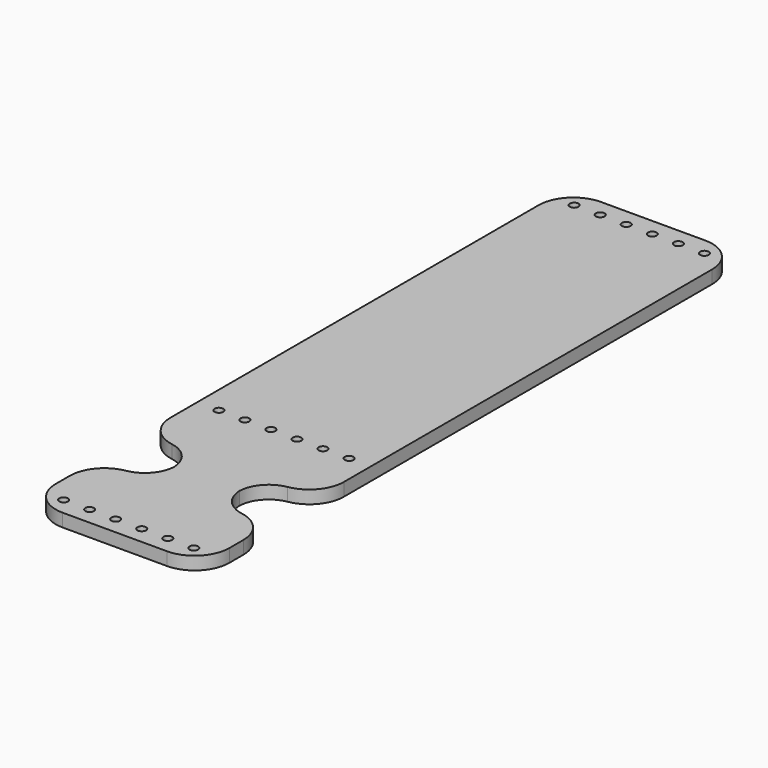
from build123d import *

# Parameters (mm, degrees)
F0_W        = 40
F0_H        = 155
F1_DEPTH    = 3
F2_W        = 12.5
F2_H        = 13
F3_DEPTH    = 3
F4_R        = 8
F5_T1_DEPTH = 3
F6_R        = 1
F7_DEPTH    = 3


# Not quite as in the source:
# - a fillet or chamfer that OpenCascade refuses, or shapes differently, is made with other operations: its cross-section is extruded or revolved along the edge and cut away or added


with BuildPart() as f1:
    # F0 (on Top) → F1 (new body)
    with BuildSketch(Plane.XY):
        Rectangle(F0_W, F0_H)
    extrude(amount=F1_DEPTH)

    # F2 (on face) → F3 (cut, through all)
    with BuildSketch(Plane.XY.offset(3)):
        with Locations((-13.75, -51)):
            Rectangle(F2_W, F2_H)
        with Locations((13.75, -51)):
            Rectangle(F2_W, F2_H)
    extrude(amount=-F3_DEPTH, mode=Mode.SUBTRACT)

    # F4
    f4_edges = [f1.edges().sort_by_distance(p)[0] for p in [
        (-20, -44.5, 1.5),
        (20, -44.5, 1.5),
        (20, -57.5, 1.5),
        (-20, -57.5, 1.5),
        (-20, -77.5, 1.5),
        (20, -77.5, 1.5),
        (-20, 77.5, 1.5),
        (20, 77.5, 1.5),
    ]]
    fillet(f4_edges, radius=F4_R)

    # F5: fillet of radius 7 on 4 edges, made by hand

    # F5_s2 → F5_t1 (join)
    with BuildSketch(Plane.XY):
        with BuildLine():
            ThreePointArc((-13.3333333333, -44.3881063775), (-9.1536616892, -46.7717188872), (-7.5, -51.2901994578))
            Line((-7.5, -51.2901994578), (-6.8, -51.2901994578))
            Line((-6.8, -51.2901994578), (-6.8, -44.5))
            Line((-6.8, -44.5), (-7.5, -43.8))
            ThreePointArc((-7.5, -43.8), (-12, -43.8), (-13.2166666667, -43.6978970694))
            Line((-13.2166666667, -43.6978970694), (-13.3333333333, -44.3881063775))
        make_face()
        with BuildLine():
            ThreePointArc((-7.5, -50.7098005422), (-9.1536616892, -55.2282811128), (-13.3333333333, -57.6118936225))
            Line((-13.3333333333, -57.6118936225), (-13.2166666667, -58.3021029306))
            ThreePointArc((-13.2166666667, -58.3021029306), (-12, -58.2), (-7.5, -58.2))
            Line((-7.5, -58.2), (-6.8, -57.5))
            Line((-6.8, -57.5), (-6.8, -50.7098005422))
            Line((-6.8, -50.7098005422), (-7.5, -50.7098005422))
        make_face()
        with BuildLine():
            ThreePointArc((13.3333333333, -44.3881063775), (9.1536616892, -46.7717188872), (7.5, -51.2901994578))
            Line((7.5, -51.2901994578), (6.8, -51.2901994578))
            Line((6.8, -51.2901994578), (6.8, -44.5))
            Line((6.8, -44.5), (7.5, -43.8))
            ThreePointArc((7.5, -43.8), (12, -43.8), (13.2166666667, -43.6978970694))
            Line((13.2166666667, -43.6978970694), (13.3333333333, -44.3881063775))
        make_face()
        with BuildLine():
            ThreePointArc((7.5, -50.7098005422), (9.1536616892, -55.2282811128), (13.3333333333, -57.6118936225))
            Line((13.3333333333, -57.6118936225), (13.2166666667, -58.3021029306))
            ThreePointArc((13.2166666667, -58.3021029306), (12, -58.2), (7.5, -58.2))
            Line((7.5, -58.2), (6.8, -57.5))
            Line((6.8, -57.5), (6.8, -50.7098005422))
            Line((6.8, -50.7098005422), (7.5, -50.7098005422))
        make_face()
    extrude(amount=F5_T1_DEPTH)

    # F6 (on face) → F7 (cut, through all)
    with BuildSketch(Plane.XY.offset(3)):
        with Locations((-15, -73.5)):
            Circle(F6_R)
        with Locations((-9, -73.5)):
            Circle(F6_R)
        with Locations((-3, -73.5)):
            Circle(F6_R)
        with Locations((3, -73.5)):
            Circle(F6_R)
        with Locations((-15, -28.8)):
            Circle(F6_R)
        with Locations((-9, -28.8)):
            Circle(F6_R)
        with Locations((-3, -28.8)):
            Circle(F6_R)
        with Locations((3, -28.8)):
            Circle(F6_R)
        with Locations((-15, 73.5)):
            Circle(F6_R)
        with Locations((-9, 73.5)):
            Circle(F6_R)
        with Locations((-3, 73.5)):
            Circle(F6_R)
        with Locations((3, 73.5)):
            Circle(F6_R)
        with Locations((9, -73.5)):
            Circle(F6_R)
        with Locations((15, -73.5)):
            Circle(F6_R)
        with Locations((9, -28.8)):
            Circle(F6_R)
        with Locations((15, -28.8)):
            Circle(F6_R)
        with Locations((9, 73.5)):
            Circle(F6_R)
        with Locations((15, 73.5)):
            Circle(F6_R)
    extrude(amount=-F7_DEPTH, mode=Mode.SUBTRACT)


solid = f1.part
